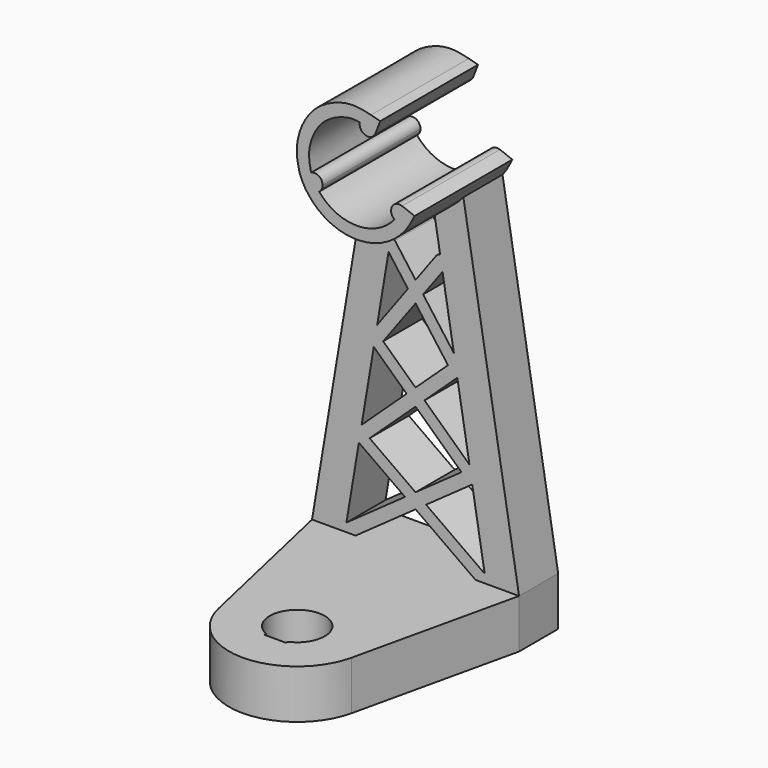
from build123d import *

# Parameters (mm, degrees)
F2_DEPTH  = 6
F3_DEPTH  = 15
F4_DEPTH  = 35
F6_DEPTH  = 6
F8_D      = 6.7564
F10_DEPTH = 6


# Not quite as in the source:
# - the dataset's text gives a spline's control points without its knots; the knots are read off the source's solid
# - a feature names something its author has since deleted; it is built from what else it names


with BuildPart() as f2:
    # F1 (on Front) → F2 (new body)
    with BuildSketch(Plane.XZ):
        with BuildLine():
            Line((8.6542004719, 6), (12.7, 6))
            Line((12.7, 6), (5.8705407632, 46.857372))
            ThreePointArc((5.8705407633, 46.857372), (4.2424830958, 45.3402334578), (2.2409148691, 44.3676051842))
            Line((2.2409148691, 44.3676051842), (8.6542004719, 6))
        make_face()
    extrude(amount=F2_DEPTH)



with BuildPart() as f2b:
    # F1 (on Front) → F2, piece 2 (new body)
    with BuildSketch(Plane.XZ):
        with BuildLine():
            Line((-5.8705407632, 46.857372), (-12.7, 6))
            Line((-12.7, 6), (-8.6542004719, 6))
            Line((-8.6542004719, 6), (-2.2409148691, 44.3676051842))
            ThreePointArc((-2.2409148691, 44.3676051842), (-4.2424830958, 45.3402334578), (-5.8705407633, 46.857372))
        make_face()
    extrude(amount=F2_DEPTH)


with BuildPart() as f2_1:
    add(f2.part)

    add(f2b.part)  # F3 merges F2b
    # F1 (on Front) → F3 (join)
    with BuildSketch(Plane.XZ):
        with BuildLine():
            ThreePointArc((2.2409148691, 44.3676051842), (4.2424830958, 45.3402334578), (5.8705407633, 46.857372))
            ThreePointArc((5.8705407633, 46.857372), (6.282563949, 47.4287346001), (6.6391644971, 48.0362330573))
            Line((6.6391644971, 48.0362330573), (7.0807542652, 48.8765835762))
            Line((7.0807542652, 48.8765835762), (5.5524562219, 49.4593701636))
            ThreePointArc((5.5524562219, 49.4593701636), (6.0196522099, 49.0923165787), (6.1961524227, 48.525))
            ThreePointArc((6.1961524227, 48.525), (5.6596016389, 47.6388765188), (4.6257227748, 47.7036535343))
            ThreePointArc((4.6257227748, 47.7036535343), (0, 45.525), (-4.6257227748, 47.7036535343))
            ThreePointArc((-4.6257227748, 47.7036535343), (-6.0645272665, 48.0290916105), (-5.6136887823, 49.4336602162))
            add(Edge.make_bspline(
                [(-5.6136887823, 49.4336602162), (-5.6731088448, 49.6796237872), (-5.7820596183, 50.1939122872), (-5.870383513, 50.9082459696), (-5.8711604748, 51.6118292097), (-5.7737215398, 52.3201730378), (-5.5545798743, 53.0961789846), (-5.2190384449, 53.8768861037), (-4.8540013097, 54.4868265304), (-4.5203343404, 54.92669058), (-4.2529215633, 55.2269683884), (-3.9690505528, 55.4953654214), (-3.551365623, 55.8301037709), (-2.9760248577, 56.1929485464), (-2.3670271983, 56.4737978906), (-1.8885428143, 56.6453539404), (-1.540980473, 56.7473331473), (-1.2165318351, 56.8219773781), (-0.927008256, 56.8678653475), (-0.6459300873, 56.8904215461), (-0.2552435271, 56.890659975), (0.0932697855, 56.8542282174), (0.3683018095, 56.8082372577)],
                knots=[0.0108020561, 0.0108020561, 0.0108020561, 0.0108020561, 0.0625, 0.125, 0.1875, 0.25, 0.3125, 0.375, 0.4375, 0.46875, 0.5, 0.53125, 0.5625, 0.625, 0.6875, 0.71875, 0.75, 0.78125, 0.8125, 0.84375, 0.875, 0.9366195247, 0.9366195247, 0.9366195247, 0.9366195247], degree=3))
            ThreePointArc((0.3683018095, 56.8082372577), (0.8230918758, 57.451680428), (1.6026947124, 57.5660156149))
            Line((1.6026947124, 57.5660156149), (1.7309102894, 58.049296864))
            add(Edge.make_bspline(
                [(-7.0293442287, 48.9099818903), (-7.3565832443, 50.2039835315), (-7.6193012084, 52.5374683234), (-5.6163940597, 56.7141750893), (-1.6495097654, 58.5359038971), (0.168253016, 58.439057015), (1.7309102894, 58.049296864)],
                knots=[0, 0, 0, 0, 0.2432574854, 0.5083218435, 0.7608988909, 1, 1, 1, 1], degree=3))
            ThreePointArc((-7.0293442287, 48.9099818903), (-6.5310841399, 47.8378683292), (-5.8705407633, 46.857372))
            ThreePointArc((-5.8705407633, 46.857372), (-4.2424830958, 45.3402334578), (-2.2409148691, 44.3676051842))
            ThreePointArc((-2.2409148691, 44.3676051842), (0, 44.025), (2.2409148691, 44.3676051842))
        make_face()
        with BuildLine():
            ThreePointArc((-5.6136887823, 49.4336602162), (-6.0645272665, 48.0290916105), (-4.6257227748, 47.7036535343))
            ThreePointArc((-4.6257227748, 47.7036535343), (-4.3100289415, 48.0615507838), (-4.1961524227, 48.525))
            ThreePointArc((-4.1961524227, 48.525), (-4.6564934376, 49.3668837092), (-5.6136887823, 49.4336602162))
        make_face()
        with BuildLine():
            ThreePointArc((6.1961524227, 48.525), (6.0196522099, 49.0923165787), (5.5524562219, 49.4593701636))
            ThreePointArc((5.5524562219, 49.4593701636), (4.3117895501, 48.9918000745), (4.6257227748, 47.7036535343))
            ThreePointArc((4.6257227748, 47.7036535343), (5.6596016389, 47.6388765188), (6.1961524227, 48.525))
        make_face()
        with BuildLine():
            ThreePointArc((2.3462635584, 56.5994531165), (2.1388640738, 57.2091943919), (1.6026947124, 57.5660156149))
            Line((1.6026947124, 57.5660156149), (1.3462178297, 56.5992807519))
            Line((1.3462178297, 56.5992807519), (1.0898324044, 55.6328906181))
            ThreePointArc((1.0898324044, 55.6328906181), (1.8000781772, 55.7083569983), (2.2788130397, 56.2384109237))
            ThreePointArc((2.2788130397, 56.2384109237), (2.3292563054, 56.4158087336), (2.3462635584, 56.5994531165))
        make_face()
        with BuildLine():
            Line((2.8635693149, 57.7487999365), (1.7309102894, 58.049296864))
            Line((1.7309102894, 58.049296864), (1.6026947124, 57.5660156149))
            ThreePointArc((1.6026947124, 57.5660156149), (2.1388640738, 57.2091943919), (2.3462635584, 56.5994531165))
            ThreePointArc((2.3462635584, 56.5994531165), (2.3292563054, 56.4158087336), (2.2788130397, 56.2384109237))
            Line((2.2788130397, 56.2384109237), (2.8635693149, 57.7487999365))
        make_face()
        with BuildLine():
            Line((1.3462178297, 56.5992807519), (1.6026947124, 57.5660156149))
            ThreePointArc((1.6026947124, 57.5660156149), (0.8230918758, 57.451680428), (0.3683018095, 56.8082372577))
            add(Edge.make_bspline(
                [(0.3683018095, 56.8082372577), (0.3722317151, 56.8075800974), (0.6504622174, 56.7608452295), (0.9735825201, 56.6917999523), (1.3462178297, 56.5992807519)],
                knots=[0.9366195247, 0.9366195247, 0.9366195247, 0.9366195247, 0.9375, 0.9988141525, 0.9988141525, 0.9988141525, 0.9988141525], degree=3))
        make_face()
        with BuildLine():
            add(Edge.make_bspline(
                [(0.3683018095, 56.8082372577), (0.3722317151, 56.8075800974), (0.6504622174, 56.7608452295), (0.9735825201, 56.6917999523), (1.3462178297, 56.5992807519)],
                knots=[0.9366195247, 0.9366195247, 0.9366195247, 0.9366195247, 0.9375, 0.9988141525, 0.9988141525, 0.9988141525, 0.9988141525], degree=3))
            ThreePointArc((0.3683018095, 56.8082372577), (0.4940362469, 56.0762814339), (1.0898324044, 55.6328906181))
            Line((1.0898324044, 55.6328906181), (1.3462178297, 56.5992807519))
        make_face()
    extrude(amount=F3_DEPTH)

    # F1 (on Front) → F4 (join)
    with BuildSketch(Plane.XZ):
        Polygon((-12.7, 0), (12.7, 0), (12.7, 6), (8.6542004719, 6), (-8.6542004719, 6), (-12.7, 6), align=None)
    extrude(amount=F4_DEPTH)

    # F5 (on face) → F6 (join)
    with BuildSketch(Plane.XZ):
        with BuildLine():
            Line((5.6317699715, 17.0785580839), (6.3808853079, 17.6112292414))
            ThreePointArc((6.3808853079, 17.6112292414), (6.8651741942, 17.7483538533), (7.3270954081, 17.5484346776))
            Line((7.3270954081, 17.5484346776), (1.0995236247, 23.3575740521))
            Line((1.0995236247, 23.3575740521), (0, 22.3319277483))
            Line((0, 22.3319277483), (5.6317699715, 17.0785580839))
        make_face()
        with BuildLine():
            ThreePointArc((7.3270954081, 17.5484346776), (6.8651741942, 17.7483538533), (6.3808853079, 17.6112292414))
            Line((6.3808853079, 17.6112292414), (5.6317699715, 17.0785580839))
            Line((5.6317699715, 17.0785580839), (6.3039250325, 16.4515653224))
            ThreePointArc((6.3039250325, 16.4515653224), (6.7658462464, 16.2516461467), (7.2501351327, 16.3887707586))
            ThreePointArc((7.2501351327, 16.3887707586), (7.5638640736, 16.9503360261), (7.3270954081, 17.5484346776))
        make_face()
        with BuildLine():
            Line((6.3039250325, 16.4515653224), (5.6317699715, 17.0785580839))
            Line((5.6317699715, 17.0785580839), (0, 13.0739925869))
            Line((0, 13.0739925869), (1.2942194152, 12.1537159347))
            Line((1.2942194152, 12.1537159347), (7.2501351327, 16.3887707586))
            ThreePointArc((7.2501351327, 16.3887707586), (6.7658462464, 16.2516461467), (6.3039250325, 16.4515653224))
        make_face()
        with BuildLine():
            Line((0, 24.3832203559), (1.0995236247, 23.3575740521))
            Line((1.0995236247, 23.3575740521), (5.4884051564, 27.4515653224))
            ThreePointArc((5.4884051564, 27.4515653224), (4.9077119005, 27.2531907373), (4.3732819976, 27.5547563392))
            Line((4.3732819976, 27.5547563392), (3.9765285291, 28.092564745))
            Line((3.9765285291, 28.092564745), (0, 24.3832203559))
        make_face()
        Polygon((0, 22.3319277483), (1.0995236247, 23.3575740521), (0, 24.3832203559), (-1.0995236247, 23.3575740521), align=None)
        Polygon((1.2942194152, 12.1537159347), (0, 13.0739925869), (-1.2942194152, 12.1537159347), (0, 11.2334392824), align=None)
        with BuildLine():
            Line((-1.2942194152, 12.1537159347), (0, 13.0739925869))
            Line((0, 13.0739925869), (-5.6317699715, 17.0785580839))
            Line((-5.6317699715, 17.0785580839), (-6.3039250325, 16.4515653224))
            ThreePointArc((-6.3039250325, 16.4515653224), (-6.7658462464, 16.2516461467), (-7.2501351327, 16.3887707586))
            Line((-7.2501351327, 16.3887707586), (-1.2942194152, 12.1537159347))
        make_face()
        with BuildLine():
            Line((-5.6317699715, 17.0785580839), (0, 22.3319277483))
            Line((0, 22.3319277483), (-1.0995236247, 23.3575740521))
            Line((-1.0995236247, 23.3575740521), (-7.3270954081, 17.5484346776))
            ThreePointArc((-7.3270954081, 17.5484346776), (-6.8651741942, 17.7483538533), (-6.3808853079, 17.6112292414))
            Line((-6.3808853079, 17.6112292414), (-5.6317699715, 17.0785580839))
        make_face()
        with BuildLine():
            Line((9.0888253844, 6.6112292414), (1.2942194152, 12.1537159347))
            Line((1.2942194152, 12.1537159347), (0, 11.2334392824))
            Line((0, 11.2334392824), (8.2195755595, 5.3887707586))
            ThreePointArc((8.2195755595, 5.3887707586), (9.2654297133, 5.5653750876), (9.0888253844, 6.6112292414))
        make_face()
        with BuildLine():
            ThreePointArc((4.3732819976, 27.5547563392), (4.9077119005, 27.2531907373), (5.4884051564, 27.4515653224))
            ThreePointArc((5.4884051564, 27.4515653224), (5.7236292314, 27.9308919319), (5.5803579397, 28.4452436608))
            ThreePointArc((5.5803579397, 28.4452436608), (5.0459280368, 28.7468092627), (4.4652347809, 28.5484346776))
            Line((4.4652347809, 28.5484346776), (3.9765285291, 28.092564745))
            Line((3.9765285291, 28.092564745), (4.3732819976, 27.5547563392))
        make_face()
        with BuildLine():
            Line((-1.0995236247, 23.3575740521), (0, 24.3832203559))
            Line((0, 24.3832203559), (-3.9765285291, 28.092564745))
            Line((-3.9765285291, 28.092564745), (-4.3732819976, 27.5547563392))
            ThreePointArc((-4.3732819976, 27.5547563392), (-4.9077119005, 27.2531907373), (-5.4884051564, 27.4515653224))
            Line((-5.4884051564, 27.4515653224), (-1.0995236247, 23.3575740521))
        make_face()
        with BuildLine():
            Line((0, 11.2334392824), (-1.2942194152, 12.1537159347))
            Line((-1.2942194152, 12.1537159347), (-9.0888253844, 6.6112292414))
            ThreePointArc((-9.0888253844, 6.6112292414), (-9.2654297133, 5.5653750876), (-8.2195755595, 5.3887707586))
            Line((-8.2195755595, 5.3887707586), (0, 11.2334392824))
        make_face()
        with BuildLine():
            Line((-6.3039250325, 16.4515653224), (-5.6317699715, 17.0785580839))
            Line((-5.6317699715, 17.0785580839), (-6.3808853079, 17.6112292414))
            ThreePointArc((-6.3808853079, 17.6112292414), (-6.8651741942, 17.7483538533), (-7.3270954081, 17.5484346776))
            ThreePointArc((-7.3270954081, 17.5484346776), (-7.5638640736, 16.9503360261), (-7.2501351327, 16.3887707586))
            ThreePointArc((-7.2501351327, 16.3887707586), (-6.7658462464, 16.2516461467), (-6.3039250325, 16.4515653224))
        make_face()
        with BuildLine():
            ThreePointArc((4.4652347809, 28.5484346776), (5.0459280368, 28.7468092627), (5.5803579397, 28.4452436608))
            Line((5.5803579397, 28.4452436608), (0.9320043261, 34.7461933562))
            Line((0.9320043261, 34.7461933562), (0, 33.4828401644))
            Line((0, 33.4828401644), (3.9765285291, 28.092564745))
            Line((3.9765285291, 28.092564745), (4.4652347809, 28.5484346776))
        make_face()
        with BuildLine():
            Line((-4.3732819976, 27.5547563392), (-3.9765285291, 28.092564745))
            Line((-3.9765285291, 28.092564745), (0, 33.4828401644))
            Line((0, 33.4828401644), (-0.9320043261, 34.7461933562))
            Line((-0.9320043261, 34.7461933562), (-5.5803579397, 28.4452436608))
            ThreePointArc((-5.5803579397, 28.4452436608), (-5.7236292314, 27.9308919319), (-5.4884051564, 27.4515653224))
            ThreePointArc((-5.4884051564, 27.4515653224), (-4.9077119005, 27.2531907373), (-4.3732819976, 27.5547563392))
        make_face()
        with BuildLine():
            Line((0, 36.009546548), (0.9320043261, 34.7461933562))
            Line((0.9320043261, 34.7461933562), (3.7416676881, 38.5547563392))
            ThreePointArc((3.7416676881, 38.5547563392), (3.5833733778, 39.6035379711), (2.5345917459, 39.4452436608))
            Line((2.5345917459, 39.4452436608), (0, 36.009546548))
        make_face()
        Polygon((0, 33.4828401644), (0.9320043261, 34.7461933562), (0, 36.009546548), (-0.9320043261, 34.7461933562), align=None)
        with BuildLine():
            Line((-0.9320043261, 34.7461933562), (0, 36.009546548))
            Line((0, 36.009546548), (-2.5345917459, 39.4452436608))
            ThreePointArc((-2.5345917459, 39.4452436608), (-3.5833733778, 39.6035379711), (-3.7416676881, 38.5547563392))
            Line((-3.7416676881, 38.5547563392), (-0.9320043261, 34.7461933562))
        make_face()
    extrude(amount=F6_DEPTH)

    # F8 (through all)
    with Locations(Plane.XY.offset(6)):
        with Locations((0, -24.1493210196)):
            Hole(F8_D / 2)

    # F9 (on face) → F10 (cut, through all)
    with BuildSketch(Plane.XY.offset(6)):
        with BuildLine():
            ThreePointArc((8.1713298888, -25.9996191278), (0, -32.5275210196), (-8.1713298888, -25.9996191278))
            Line((-8.1713298888, -25.9996191278), (-12.7, -6))
            Line((-12.7, -6), (-12.7, -35))
            Line((-12.7, -35), (12.7, -35))
            Line((12.7, -35), (12.7, -6))
            Line((12.7, -6), (8.1713298888, -25.9996191278))
        make_face()
        with BuildLine():
            Line((1.3396433368, -27.5275210196), (1.3396433368, -27.250545128))
            ThreePointArc((1.3396433368, -27.250545128), (0.6839882883, -27.4575524598), (0, -27.5275210196))
            Line((0, -27.5275210196), (1.3396433368, -27.5275210196))
        make_face()
        with BuildLine():
            ThreePointArc((0, -27.5275210196), (-0.6839882883, -27.4575524598), (-1.3396433368, -27.250545128))
            Line((-1.3396433368, -27.250545128), (-1.3396433368, -27.5275210196))
            Line((-1.3396433368, -27.5275210196), (0, -27.5275210196))
        make_face()
    extrude(amount=-F10_DEPTH, mode=Mode.SUBTRACT)


solid = f2_1.part
